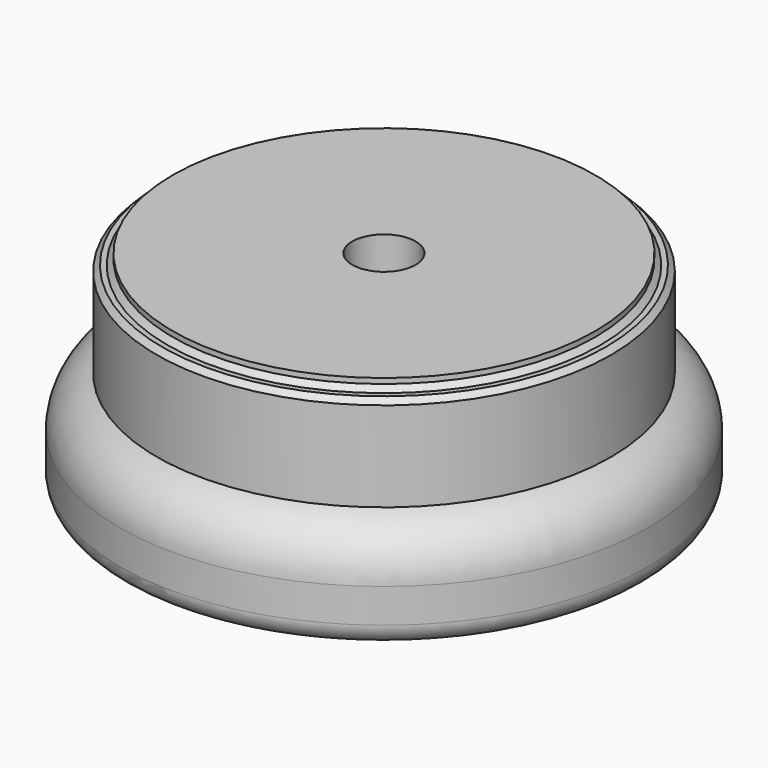
from build123d import *

# Parameters (mm, degrees)
F3_R     = 2
F4_SIZE  = 0.5
F5_R     = 3
F6_DEPTH = 20.001


# Not quite as in the source:
# - a fillet or chamfer that OpenCascade refuses, or shapes differently, is made with other operations: its cross-section is extruded or revolved along the edge and cut away or added


with BuildPart() as f1:
    # F0 (on Front) → F1 (revolve)
    with BuildSketch(Plane.XZ):
        Polygon((0, 20), (0, 0), (25, 0), (25, 10), (21.5, 10), (21.5, 19), (20, 19), (20, 20), align=None)
    revolve(axis=Axis((0, 0, 11.1239180034), (0, 0, -1)))

    # F2: fillet of radius 5 on 1 edges, made by hand

    # F2_s1 → F2_t2 (revolve, cut)
    with BuildSketch(Plane.XZ):
        with BuildLine():
            ThreePointArc((25, 5.2303039929), (24.0311288741, 8.1883438845), (21.5, 10))
            Line((21.5, 10), (25, 10))
            Line((25, 10), (25, 5.2303039929))
        make_face()
    revolve(axis=Axis((0, 0, 10), (0, 0, -1)), mode=Mode.SUBTRACT)

    # F3
    f3_edges = [f1.edges().sort_by_distance(p)[0] for p in [
        (-25, 0, 0),
    ]]
    fillet(f3_edges, radius=F3_R)

    # F4
    f4_edges = [f1.edges().sort_by_distance(p)[0] for p in [
        (-21.5, 0, 19),
        (-20, 0, 19),
    ]]
    chamfer(f4_edges, length=F4_SIZE)

    # F5 (on face) → F6 (cut, through all)
    with BuildSketch(Plane.XY.offset(20)):
        Circle(F5_R)
    extrude(amount=-F6_DEPTH, mode=Mode.SUBTRACT)


solid = f1.part
